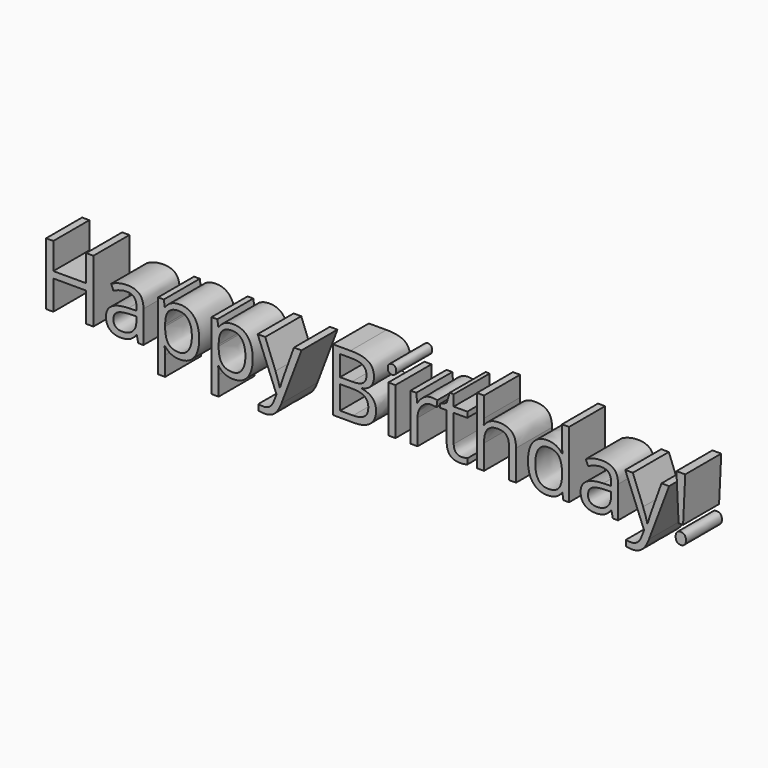
from build123d import *

# Parameters (mm, degrees)
F0_TEXT_SIZE = 49.3005665097
F1_DEPTH     = 25.4


# Not quite as in the source:
# - Text() gives the source's letters only with a copy of the font that has no kerning and outlines rounded to 1/6400 em; it was checked with that copy


with BuildPart() as f1:
    # F0 (on Front) → F1 (new body)
    with BuildSketch(Plane.XZ):
        with Locations((-30.3499605507, -3.7428082433)):
            Text('Happy Birthday!', F0_TEXT_SIZE, font='Open Sans', text_align=(TextAlign.LEFT, TextAlign.BOTTOM))
    extrude(amount=F1_DEPTH)


solid = f1.part
